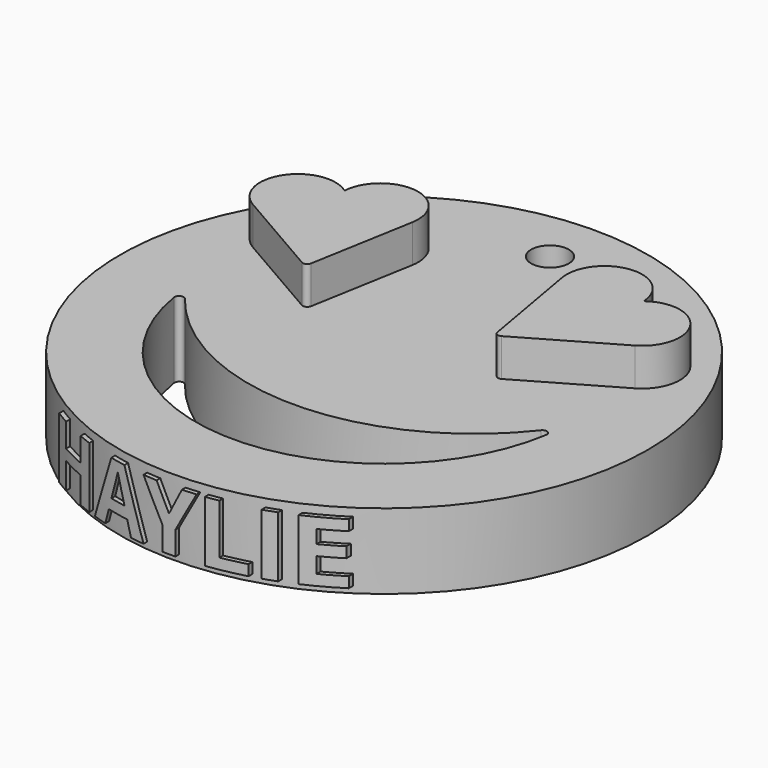
from build123d import *

# Parameters (mm, degrees)
F0_R         = 22.225
F1_DEPTH     = 6.35
F3_DEPTH     = 3.175
F4_R         = 1.5875
F5_DEPTH     = 6.351
F6_R         = 0.381
F8_TEXT_SIZE = 7.172925032
F9_DEPTH     = 4.445
F11_DEPTH    = 6.3510001


# Not quite as in the source:
# - Text() gives the source's letters only with a copy of the font that has no kerning and outlines rounded to 1/6400 em; it was checked with that copy


with BuildPart() as f1:
    # F0 (on Top) → F1 (new body)
    with BuildSketch(Plane.XY):
        Circle(F0_R)
    extrude(amount=F1_DEPTH)

    # F2 (on face) → F3 (join)
    with BuildSketch(Plane.XY.offset(6.35)):
        with BuildLine():
            Line((-16.0822255904, 6.2898595121), (-7.9375, 1.5875))
            Line((-7.9375, 1.5875), (-6.30438768, 10.8493402099))
            ThreePointArc((-6.30438768, 10.8493402099), (-9.0613841419, 14.5540676168), (-12.6006424639, 11.5876412851))
            ThreePointArc((-12.6006424639, 11.5876412851), (-17.1480482681, 10.7831942059), (-16.0822255904, 6.2898595121))
        make_face()
        with BuildLine():
            ThreePointArc((16.0822255904, 6.2898595121), (17.1480482681, 10.7831942059), (12.6006424639, 11.5876412851))
            ThreePointArc((12.6006424639, 11.5876412851), (9.0613841419, 14.5540676168), (6.30438768, 10.8493402099))
            Line((6.30438768, 10.8493402099), (7.9375, 1.5875))
            Line((7.9375, 1.5875), (16.0822255904, 6.2898595121))
        make_face()
    extrude(amount=F3_DEPTH)

    # F4 (on face) → F5 (cut, through all)
    with BuildSketch(Plane.XY.offset(6.35)):
        with BuildLine():
            ThreePointArc((15.8396829373, -1.0583333333), (0, -9.525), (-15.8396829373, -1.0583333333))
            ThreePointArc((-15.8396829373, -1.0583333333), (0, -15.875), (15.8396829373, -1.0583333333))
        make_face()
        with Locations((0, 17.4625)):
            Circle(F4_R)
    extrude(amount=-F5_DEPTH, mode=Mode.SUBTRACT)

    # F6
    f6_edges = [f1.edges().sort_by_distance(p)[0] for p in [
        (-7.9375, 1.5875, 7.9375),
        (7.9375, 1.5875, 7.9375),
        (15.839683, -1.058333, 3.175),
        (-15.839683, -1.058333, 3.175),
    ]]
    fillet(f6_edges, radius=F6_R)

    # F8 (on offset) → F9 (join)
    with BuildSketch(Plane.XZ.offset(22.606)):
        with Locations((-12.7, 0.5617718408)):
            Text('HAYLIE', F8_TEXT_SIZE, font='Open Sans', font_style=FontStyle.BOLD, text_align=(TextAlign.LEFT, TextAlign.BOTTOM))
    extrude(amount=-F9_DEPTH)

    # F10 (on face) → F11 (cut, through all)
    with BuildSketch(Plane.XY.offset(6.35)):
        with BuildLine():
            ThreePointArc((16.2992915562, -15.6641096385), (2.0819108343, -22.5099285489), (-13.1498776067, -18.3878208315))
            Line((-13.1498776067, -18.3878208315), (-13.1498776067, -35.9964779015))
            Line((-13.1498776067, -35.9964779015), (16.2992915562, -35.9964779015))
            Line((16.2992915562, -35.9964779015), (16.2992915562, -15.6641096385))
        make_face()
    extrude(amount=-F11_DEPTH, mode=Mode.SUBTRACT)


solid = f1.part
